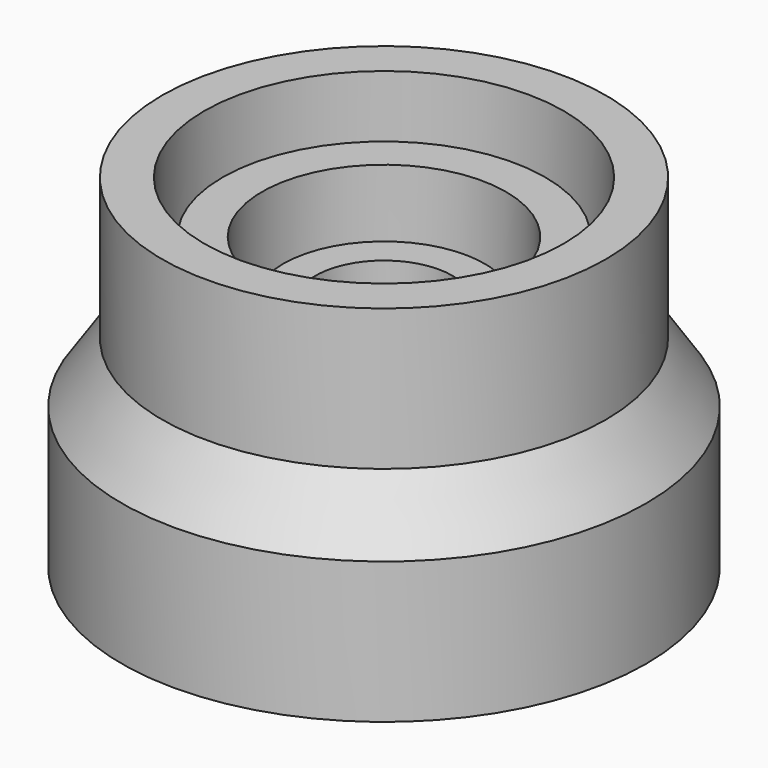
from build123d import *

# Parameters (mm, degrees)
F2_R      = 17
F4_DEPTH  = 58.001
F3_R      = 30.25
F5_DEPTH  = 30
F8_R      = 30.25
F9_DEPTH  = 72.001
F10_R     = 44.55
F10_R_2   = 30.25
F11_DEPTH = 30
F14_R     = 44.55
F15_DEPTH = 85.001
F16_R     = 57.15
F16_R_2   = 44.55
F17_DEPTH = 35


with BuildPart() as f1:
    # F0 (on Front) → F1 (revolve)
    with BuildSketch(Plane.XZ):
        Polygon((-40, 0), (0, 0), (0, 58), (-25, 58), (-25, 43), (-40, 30), align=None)
    revolve(axis=Axis((0, 0, 29), (0, 0, 1)))

    # F2 (on face) → F4 (cut, through all)
    with BuildSketch(Plane.XY.offset(58)):
        Circle(F2_R)
    extrude(amount=-F4_DEPTH, mode=Mode.SUBTRACT)

    # F3 (on face) → F5 (cut)
    with BuildSketch(Plane(origin=(0, 0, 0), x_dir=(1, 0, 0), z_dir=(0, 0, -1))):
        Circle(F3_R)
    extrude(amount=-F5_DEPTH, mode=Mode.SUBTRACT)


with BuildPart() as f7:
    # F6 (on Front) → F7 (revolve)
    with BuildSketch(Plane.XZ):
        Polygon((-55, 0), (0, 0), (0, 72), (-40, 72), (-40, 47), (-55, 35), align=None)
    revolve(axis=Axis((0, 0, 36), (0, 0, 1)))

    # F8 (on face) → F9 (cut, through all)
    with BuildSketch(Plane.XY.offset(72)):
        Circle(F8_R)
    extrude(amount=-F9_DEPTH, mode=Mode.SUBTRACT)

    # F10 (on face) → F11 (cut)
    with BuildSketch(Plane(origin=(0, 0, 0), x_dir=(1, 0, 0), z_dir=(0, 0, -1))):
        Circle(F10_R)
        Circle(F10_R_2, mode=Mode.SUBTRACT)
    extrude(amount=-F11_DEPTH, mode=Mode.SUBTRACT)


with BuildPart() as f13:
    # F12 (on Front) → F13 (revolve)
    with BuildSketch(Plane.XZ):
        Polygon((-65, 0), (0, 0), (0, 85), (-55, 85), (-55, 50), (-65, 35), align=None)
    revolve(axis=Axis((0, 0, 42.5), (0, 0, 1)))

    # F14 (on face) → F15 (cut, through all)
    with BuildSketch(Plane.XY.offset(85)):
        Circle(F14_R)
    extrude(amount=-F15_DEPTH, mode=Mode.SUBTRACT)

    # F16 (on face) → F17 (cut)
    with BuildSketch(Plane(origin=(0, 0, 0), x_dir=(1, 0, 0), z_dir=(0, 0, -1))):
        Circle(F16_R)
        Circle(F16_R_2, mode=Mode.SUBTRACT)
    extrude(amount=-F17_DEPTH, mode=Mode.SUBTRACT)


solid = Compound([f1.part, f7.part, f13.part])
